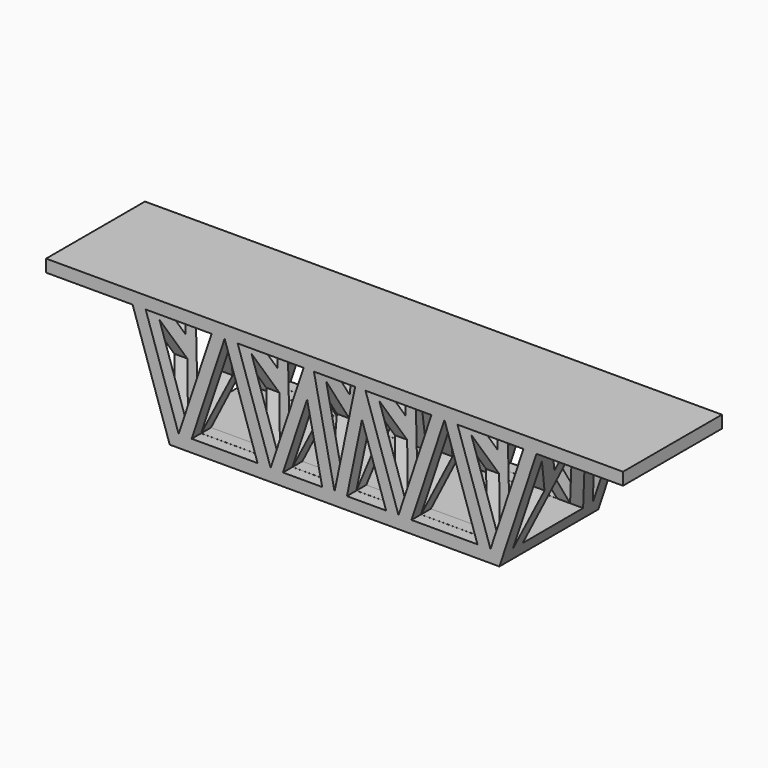
from build123d import *

# Parameters (mm, degrees)
F1_DEPTH  = 19.05
F3_DEPTH  = 64.77
F5_DEPTH  = 38.101
F7_DEPTH  = 71.628
F9_DEPTH  = 63.5
F10_W     = 177.8
F10_H     = 3.81
F11_DEPTH = 19.05


# Not quite as in the source:
# - a feature names something its author has since deleted; it is built from what else it names


with BuildPart() as f1:
    # F0 (on Front) → F1 (new body, symmetric)
    with BuildSketch(Plane.XZ):
        Polygon((63.5, 0), (-63.5, 0), (-50.8, -38.1), (50.8, -38.1), align=None)
    extrude(amount=F1_DEPTH, both=True)

    # F2 (on Right) → F3 (join, symmetric)
    with BuildSketch(Plane.YZ):
        Polygon((-13.8531752413, -2.1771209331), (-17.2030024947, -3.9922675862), (-9.4392557284, -19.4210141376), (-6.0894284749, -17.6058674845), align=None)
        Polygon((9.3579589429, -19.3780629918), (17.1217057092, -3.9493164404), (13.7183057347, -2.2367252419), (5.9545589683, -17.6654717934), align=None)
    extrude(amount=F3_DEPTH, both=True)

    # F4 (on face) → F5 (cut, through all)
    with BuildSketch(Plane.XZ.offset(19.05)):
        Polygon((19.7017221148, -34.29), (29.8617221148, -3.81), (9.5417221148, -3.81), align=None)
        Polygon((44.0378147432, -34.29), (33.8778147432, -3.81), (23.7178147432, -34.29), align=None)
        Polygon((37.8939073716, -3.81), (48.0539073716, -34.29), (58.2139073716, -3.81), align=None)
        Polygon((-9.5417221148, -3.81), (-29.8617221148, -3.81), (-19.7017221148, -34.29), align=None)
        Polygon((-23.7178147432, -34.29), (-33.8778147432, -3.81), (-44.0378147432, -34.29), align=None)
        Polygon((-37.8939073716, -3.81), (-58.2139073716, -3.81), (-48.0539073716, -34.29), align=None)
        Polygon((-8.456816198, -11.9852822497), (-15.8917221148, -34.29), (-3.81, -34.29), align=None)
        Polygon((6.35, -3.81), (0, -3.81), (-6.35, -3.81), (0, -34.29), align=None)
        Polygon((8.456816198, -11.9852822497), (3.81, -34.29), (15.8917221148, -34.29), align=None)
    extrude(amount=-F5_DEPTH, mode=Mode.SUBTRACT)

    # F6 (on Right) → F7 (cut, symmetric)
    with BuildSketch(Plane.YZ):
        Polygon((11.6265764875, -34.3226165375), (0, -3.81), (-11.6078330565, -34.356936069), align=None)
        Polygon((7.7041713773, -14.18850027), (12.8517927524, -3.9587300405), (3.8070123771, -3.9608534399), align=None)
        Polygon((15.3426150913, -34.3226165375), (15.4205774713, -7.3299362912), (9.5230814997, -19.0499180696), align=None)
        Polygon((-7.9282270394, -13.9516580075), (-3.8043182587, -4.0179966015), (-12.9268464257, -4.0179966015), align=None)
        Polygon((-9.4793978932, -19.3412403755), (-15.3408200295, -7.6929474451), (-15.4178330565, -34.356936069), align=None)
    extrude(amount=F7_DEPTH, both=True, mode=Mode.SUBTRACT)

    # F8 (on Front) → F9 (cut, symmetric)
    with BuildSketch(Plane.XZ):
        Polygon((71.0988326841, 0), (63.5, 0), (50.6969301873, -38.4092094382), (71.0988326841, -38.4092094382), align=None)
        Polygon((-50.9874074378, -37.5377776867), (-63.5, 0), (-69.8199345388, 0), (-69.8199345388, -37.5377776867), align=None)
    extrude(amount=F9_DEPTH, both=True, mode=Mode.SUBTRACT)

    # F10 (on Front) → F11 (join, symmetric)
    with BuildSketch(Plane.XZ):
        with Locations((0, -1.905)):
            Rectangle(F10_W, F10_H)
    extrude(amount=F11_DEPTH, both=True)


solid = f1.part
